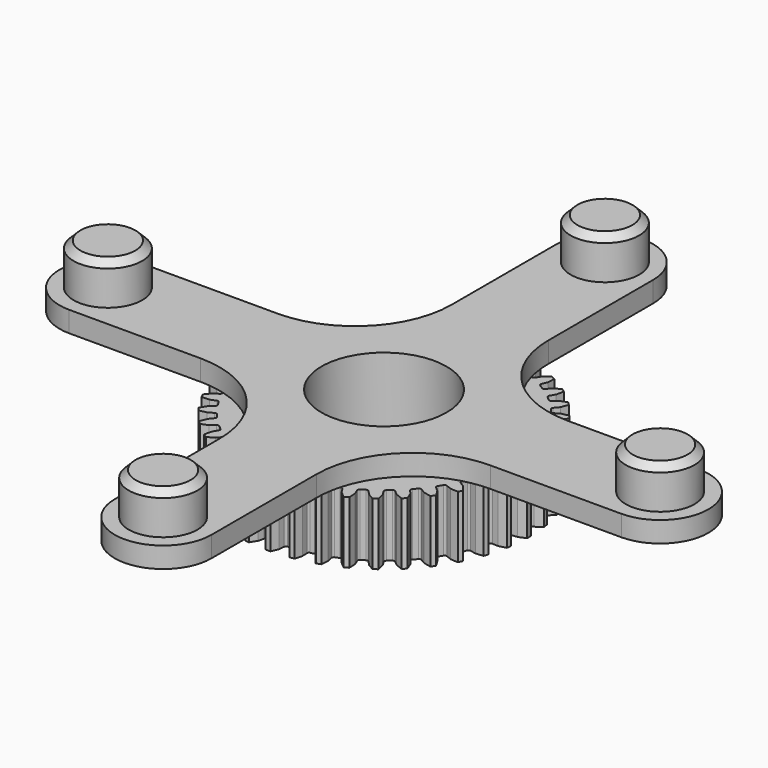
from build123d import *
from build123d import SkipClean  # not in build123d's __all__

# Parameters (mm, degrees)
F0_R     = 4.975
F0_R_2   = 14
F0_R_3   = 1
F0_R_4   = 5
F1_DEPTH = 3
F2_DEPTH = 9
F3_SIZE  = 1
F5_DEPTH = 9
F6_R     = 9.05
F6_R_2   = 5
F7_DEPTH = 18.001


# Not quite as in the source:
# - ends of sketch curves that miss each other by under 0.0002 mm in the source are joined


with BuildPart() as f1:
    # F0 (on Top) → F1 (new body)
    with BuildSketch(Plane.XY):
        with BuildLine():
            ThreePointArc((7, 40.000000175), (-1.75e-07, 47), (-7, 39.999999825))
            Line((-7, 39.999999825), (-6.999999525, 20.9999983))
            ThreePointArc((-6.999999525, 20.9999983), (-11.1005042172, 11.1005033846), (-20.999998825, 6.99999795))
            Line((-20.999998825, 6.99999795), (-40.00000035, 6.999997))
            ThreePointArc((-40.00000035, 6.999997), (-47, -3.35e-06), (-39.99999965, -7.000003))
            Line((-39.99999965, -7.000003), (-20.999999175, -7.00000205))
            ThreePointArc((-20.999999175, -7.00000205), (-11.1005039096, -11.1005067422), (-6.999998475, -21.0000017))
            Line((-6.999998475, -21.0000017), (-6.999998, -40.000000175))
            ThreePointArc((-6.999998, -40.000000175), (2.175e-06, -47), (7.000002, -39.999999825))
            Line((7.000002, -39.999999825), (7.000001525, -21.0000003))
            ThreePointArc((7.000001525, -21.0000003), (11.1005062172, -11.1005053846), (21.000000825, -6.99999995))
            Line((21.000000825, -6.99999995), (40.00000035, -6.999999))
            ThreePointArc((40.00000035, -6.999999), (47, 1.35e-06), (39.99999965, 7.000001))
            Line((39.99999965, 7.000001), (21.000001175, 7.00000005))
            ThreePointArc((21.000001175, 7.00000005), (11.1005059096, 11.1005047422), (7.000000475, 20.9999997))
            Line((7.000000475, 20.9999997), (7, 40.000000175))
        make_face()
        with Locations((-40, -3e-06)):
            Circle(F0_R, mode=Mode.SUBTRACT)
        with Locations((2e-06, -40)):
            Circle(F0_R, mode=Mode.SUBTRACT)
        Circle(F0_R_2, mode=Mode.SUBTRACT)
        with Locations((40, 1e-06)):
            Circle(F0_R, mode=Mode.SUBTRACT)
        with Locations((0, 40)):
            Circle(F0_R, mode=Mode.SUBTRACT)
        with Locations((-40, -3e-06)):
            Circle(F0_R)
        with Locations((-40, -3e-06)):
            Circle(F0_R_3, mode=Mode.SUBTRACT)
        Circle(F0_R_2)
        Circle(F0_R_4, mode=Mode.SUBTRACT)
        with Locations((40, 1e-06)):
            Circle(F0_R)
        with Locations((40, 1e-06)):
            Circle(F0_R_3, mode=Mode.SUBTRACT)
        with Locations((0, 40)):
            Circle(F0_R)
        with Locations((0, 40)):
            Circle(F0_R_3, mode=Mode.SUBTRACT)
        with Locations((2e-06, -40)):
            Circle(F0_R)
        with Locations((2e-06, -40)):
            Circle(F0_R_3, mode=Mode.SUBTRACT)
        with Locations((-40, -3e-06)):
            Circle(F0_R_3)
        with Locations((2e-06, -40)):
            Circle(F0_R_3)
        with Locations((40, 1e-06)):
            Circle(F0_R_3)
        with Locations((0, 40)):
            Circle(F0_R_3)
    extrude(amount=F1_DEPTH)

    # F0 (on Top) → F2 (join)
    with BuildSketch(Plane.XY):
        with Locations((-40, -3e-06)):
            Circle(F0_R)
        with Locations((-40, -3e-06)):
            Circle(F0_R_3, mode=Mode.SUBTRACT)
        with Locations((2e-06, -40)):
            Circle(F0_R)
        with Locations((2e-06, -40)):
            Circle(F0_R_3, mode=Mode.SUBTRACT)
        with Locations((40, 1e-06)):
            Circle(F0_R)
        with Locations((40, 1e-06)):
            Circle(F0_R_3, mode=Mode.SUBTRACT)
        with Locations((0, 40)):
            Circle(F0_R)
        with Locations((0, 40)):
            Circle(F0_R_3, mode=Mode.SUBTRACT)
        with Locations((-40, -3e-06)):
            Circle(F0_R_3)
        with Locations((2e-06, -40)):
            Circle(F0_R_3)
        with Locations((40, 1e-06)):
            Circle(F0_R_3)
        with Locations((0, 40)):
            Circle(F0_R_3)
    extrude(amount=F2_DEPTH)

    # F3
    f3_edges = [f1.edges().sort_by_distance(p)[0] for p in [
        (-44.975, -3e-06, 9),
        (-4.975, 40, 9),
        (35.025, 1e-06, 9),
        (-4.974998, -40, 9),
    ]]
    chamfer(f3_edges, length=F3_SIZE)

    # F4 (on face) → F5 (join)
    with BuildSketch(Plane(origin=(0, 0, 0), x_dir=(1, 0, 0), z_dir=(0, 0, -1))):
        with BuildLine():
            ThreePointArc((7.482641328, 17.3556929783), (11.1005062172, 11.1005053846), (17.3556935395, 7.4826400263))
            ThreePointArc((17.3556935395, 7.4826400263), (17.3405703168, 7.5176207065), (17.3253765901, 7.5525708213))
            ThreePointArc((17.3253765901, 7.5525708213), (17.313509364, 7.760210144), (17.4395229912, 7.9256730139))
            Line((17.4395229912, 7.9256730139), (18.158589, 8.38246))
            Line((18.158589, 8.38246), (18.860183, 9.235448))
            ThreePointArc((18.860183, 9.235448), (18.7111361006, 9.5338022753), (18.557366741, 9.8297578628))
            Line((18.557366741, 9.8297578628), (17.454904, 9.763521))
            Line((17.454904, 9.763521), (16.662699, 9.450277))
            ThreePointArc((16.662699, 9.450277), (16.4547675314, 9.4455858794), (16.2937556703, 9.5772398062))
            ThreePointArc((16.2937556703, 9.5772398062), (16.1149012303, 9.8752194071), (15.9305966906, 10.1698618025))
            ThreePointArc((15.9305966906, 10.1698618025), (15.8863870736, 10.3730992199), (15.9849650752, 10.5562379148))
            Line((15.9849650752, 10.5562379148), (16.623721, 11.119888))
            Line((16.623721, 11.119888), (17.183241, 12.072126))
            ThreePointArc((17.183241, 12.072126), (16.9893574176, 12.3434895607), (16.7911900572, 12.6117380429))
            Line((16.7911900572, 12.6117380429), (15.712654, 12.373864))
            Line((15.712654, 12.373864), (14.979205, 11.940548))
            ThreePointArc((14.979205, 11.940548), (14.7745668627, 11.903388278), (14.5949422111, 12.0082331737))
            ThreePointArc((14.5949422111, 12.0082331737), (14.3716706288, 12.2745705968), (14.1435428129, 12.5367538342))
            ThreePointArc((14.1435428129, 12.5367538342), (14.0680887526, 12.7305673443), (14.1368039213, 12.9268720651))
            Line((14.1368039213, 12.9268720651), (14.679522, 13.583506))
            Line((14.679522, 13.583506), (15.08319, 14.61155))
            ThreePointArc((15.08319, 14.61155), (14.8492371516, 14.8492476582), (14.6115462057, 15.0831932123))
            Line((14.6115462057, 15.0831932123), (13.583506, 14.679522))
            Line((13.583506, 14.679522), (12.926872, 14.136804))
            ThreePointArc((12.926872, 14.136804), (12.7305673443, 14.0680887526), (12.5367531183, 14.1435431335))
            ThreePointArc((12.5367531183, 14.1435431335), (12.2745678752, 14.3716729533), (12.0082271073, 14.5949471304))
            ThreePointArc((12.0082271073, 14.5949471304), (11.9033883527, 14.7745664387), (11.9405484254, 14.9792037487))
            Line((11.9405484254, 14.9792037487), (12.373864, 15.712654))
            Line((12.373864, 15.712654), (12.611741, 16.791188))
            ThreePointArc((12.611741, 16.791188), (12.3434953892, 16.989353183), (12.0721337434, 17.1832356348))
            Line((12.0721337434, 17.1832356348), (11.119888, 16.623721))
            Line((11.119888, 16.623721), (10.556238, 15.984965))
            ThreePointArc((10.556238, 15.984965), (10.3730992199, 15.8863870736), (10.1698673552, 15.9305935563))
            ThreePointArc((10.1698673552, 15.9305935563), (9.8752246071, 16.1148980437), (9.5772429612, 16.293753934))
            ThreePointArc((9.5772429612, 16.293753934), (9.4455858794, 16.4547675314), (9.4502765252, 16.6626991877))
            Line((9.4502765252, 16.6626991877), (9.763521, 17.454904))
            Line((9.763521, 17.454904), (9.829749, 18.557372))
            ThreePointArc((9.829749, 18.557372), (9.5337988946, 18.7111378232), (9.2354479733, 18.8601829454))
            Line((9.2354479733, 18.8601829454), (8.38246, 18.158589))
            Line((8.38246, 18.158589), (7.925673, 17.439523))
            ThreePointArc((7.925673, 17.439523), (7.760210144, 17.313509364), (7.552564996, 17.3253789908))
            ThreePointArc((7.552564996, 17.3253789908), (7.5176153939, 17.34057262), (7.482641328, 17.3556929783))
        make_face()
        with BuildLine():
            ThreePointArc((17.3253765901, -7.5525708213), (17.3405703617, -7.5176206031), (17.3556936288, -7.4826398191))
            ThreePointArc((17.3556936288, -7.4826398191), (11.1005054382, -11.1005052136), (7.4826401704, -17.3556934774))
            ThreePointArc((7.4826401704, -17.3556934774), (7.5176148156, -17.3405728707), (7.552558906, -17.3253817843))
            ThreePointArc((7.552558906, -17.3253817843), (7.7602105823, -17.3135094981), (7.9256730139, -17.4395229912))
            Line((7.9256730139, -17.4395229912), (8.38246, -18.158589))
            Line((8.38246, -18.158589), (9.235448, -18.860183))
            ThreePointArc((9.235448, -18.860183), (9.5337988946, -18.7111378232), (9.8297452293, -18.5573734329))
            Line((9.8297452293, -18.5573734329), (9.763521, -17.454904))
            Line((9.763521, -17.454904), (9.450277, -16.662699))
            ThreePointArc((9.450277, -16.662699), (9.4455858794, -16.4547675314), (9.5772398062, -16.2937556703))
            ThreePointArc((9.5772398062, -16.2937556703), (9.8752246071, -16.1148980437), (10.169867169, -15.9305932647))
            ThreePointArc((10.169867169, -15.9305932647), (10.3730992199, -15.8863870736), (10.5562379148, -15.9849650752))
            Line((10.5562379148, -15.9849650752), (11.119888, -16.623721))
            Line((11.119888, -16.623721), (12.072126, -17.183241))
            ThreePointArc((12.072126, -17.183241), (12.3434953892, -16.989353183), (12.6117437997, -16.7911857333))
            Line((12.6117437997, -16.7911857333), (12.373864, -15.712654))
            Line((12.373864, -15.712654), (11.940548, -14.979205))
            ThreePointArc((11.940548, -14.979205), (11.9033883527, -14.7745664387), (12.0082331737, -14.5949422111))
            ThreePointArc((12.0082331737, -14.5949422111), (12.2745678752, -14.3716729533), (12.5367580597, -14.1435390674))
            ThreePointArc((12.5367580597, -14.1435390674), (12.7305673443, -14.0680887526), (12.9268720651, -14.1368039213))
            Line((12.9268720651, -14.1368039213), (13.583506, -14.679522))
            Line((13.583506, -14.679522), (14.61155, -15.08319))
            ThreePointArc((14.61155, -15.08319), (14.8492371516, -14.8492476582), (15.0831828739, -14.6115568778))
            Line((15.0831828739, -14.6115568778), (14.679522, -13.583506))
            Line((14.679522, -13.583506), (14.136804, -12.926872))
            ThreePointArc((14.136804, -12.926872), (14.0680887526, -12.7305673443), (14.1435431335, -12.5367531183))
            ThreePointArc((14.1435431335, -12.5367531183), (14.3716706288, -12.2745705968), (14.5949389946, -12.0082369956))
            ThreePointArc((14.5949389946, -12.0082369956), (14.7745668627, -11.903388278), (14.9792044899, -11.9405488634))
            Line((14.9792044899, -11.9405488634), (15.712654, -12.373864))
            Line((15.712654, -12.373864), (16.791188, -12.611741))
            ThreePointArc((16.791188, -12.611741), (16.9893574176, -12.3434895607), (17.183239779, -12.0721278447))
            Line((17.183239779, -12.0721278447), (16.623721, -11.119888))
            Line((16.623721, -11.119888), (15.984965, -10.556238))
            ThreePointArc((15.984965, -10.556238), (15.8863870736, -10.3730992199), (15.9305935563, -10.1698673552))
            ThreePointArc((15.9305935563, -10.1698673552), (16.1149012303, -9.8752194071), (16.2937568886, -9.5772379345))
            ThreePointArc((16.2937568886, -9.5772379345), (16.4547675314, -9.4455858794), (16.6626991877, -9.4502765252))
            Line((16.6626991877, -9.4502765252), (17.454904, -9.763521))
            Line((17.454904, -9.763521), (18.557372, -9.829749))
            ThreePointArc((18.557372, -9.829749), (18.7111361006, -9.5338022753), (18.8601858954, -9.2354419488))
            Line((18.8601858954, -9.2354419488), (18.158589, -8.38246))
            Line((18.158589, -8.38246), (17.439523, -7.925673))
            ThreePointArc((17.439523, -7.925673), (17.313509364, -7.760210144), (17.3253765901, -7.5525708213))
        make_face()
        with BuildLine():
            ThreePointArc((-7.5525650468, -17.3253791074), (-7.5176170317, -17.34057191), (-7.4826384548, -17.355694217))
            ThreePointArc((-7.4826384548, -17.355694217), (-11.1005042172, -11.1005033846), (-17.3556947782, -7.4826371531))
            ThreePointArc((-17.3556947782, -7.4826371531), (-17.3405721919, -7.5176163814), (-17.3253791074, -7.5525650468))
            ThreePointArc((-17.3253791074, -7.5525650468), (-17.3135094981, -7.7602105823), (-17.4395229912, -7.9256730139))
            Line((-17.4395229912, -7.9256730139), (-18.158589, -8.38246))
            Line((-18.158589, -8.38246), (-18.860183, -9.235448))
            ThreePointArc((-18.860183, -9.235448), (-18.7111345743, -9.5338052708), (-18.5573702937, -9.8297511556))
            Line((-18.5573702937, -9.8297511556), (-17.454904, -9.763521))
            Line((-17.454904, -9.763521), (-16.662699, -9.450277))
            ThreePointArc((-16.662699, -9.450277), (-16.454767939, -9.4455857391), (-16.2937561071, -9.577239063))
            ThreePointArc((-16.2937561071, -9.577239063), (-16.1148997927, -9.875221753), (-15.9305901283, -10.1698720819))
            ThreePointArc((-15.9305901283, -10.1698720819), (-15.8863870736, -10.3730992199), (-15.9849650752, -10.5562379148))
            Line((-15.9849650752, -10.5562379148), (-16.623721, -11.119888))
            Line((-16.623721, -11.119888), (-17.183241, -12.072126))
            ThreePointArc((-17.183241, -12.072126), (-16.9893616522, -12.3434837323), (-16.791194381, -12.6117322862))
            Line((-16.791194381, -12.6117322862), (-15.712654, -12.373864))
            Line((-15.712654, -12.373864), (-14.979205, -11.940548))
            ThreePointArc((-14.979205, -11.940548), (-14.7745667516, -11.9033882976), (-14.5949426148, -12.008232683))
            ThreePointArc((-14.5949426148, -12.008232683), (-14.3716752415, -12.274565196), (-14.1435470548, -12.5367490486))
            ThreePointArc((-14.1435470548, -12.5367490486), (-14.0680887526, -12.7305673443), (-14.1368039213, -12.9268720651))
            Line((-14.1368039213, -12.9268720651), (-14.679522, -13.583506))
            Line((-14.679522, -13.583506), (-15.08319, -14.61155))
            ThreePointArc((-15.08319, -14.61155), (-14.8492426589, -14.849242151), (-14.6115517997, -15.0831877932))
            Line((-14.6115517997, -15.0831877932), (-13.583506, -14.679522))
            Line((-13.583506, -14.679522), (-12.926872, -14.136804))
            ThreePointArc((-12.926872, -14.136804), (-12.7305670127, -14.0680887583), (-12.5367526219, -14.1435435735))
            ThreePointArc((-12.5367526219, -14.1435435735), (-12.2745657312, -14.3716747845), (-12.0082320514, -14.5949430625))
            ThreePointArc((-12.0082320514, -14.5949430625), (-11.903388278, -14.7745668627), (-11.9405488634, -14.9792044899))
            Line((-11.9405488634, -14.9792044899), (-12.373864, -15.712654))
            Line((-12.373864, -15.712654), (-12.611741, -16.791188))
            ThreePointArc((-12.611741, -16.791188), (-12.3434840557, -16.9893614172), (-12.072121946, -17.1832439231))
            Line((-12.072121946, -17.1832439231), (-11.119888, -16.623721))
            Line((-11.119888, -16.623721), (-10.556238, -15.984965))
            ThreePointArc((-10.556238, -15.984965), (-10.3730992199, -15.8863870736), (-10.1698673552, -15.9305935563))
            ThreePointArc((-10.1698673552, -15.9305935563), (-9.8752221123, -16.1148995725), (-9.5772321646, -16.2937602801))
            ThreePointArc((-9.5772321646, -16.2937602801), (-9.4455857391, -16.454767939), (-9.4502765252, -16.6626991877))
            Line((-9.4502765252, -16.6626991877), (-9.763521, -17.454904))
            Line((-9.763521, -17.454904), (-9.829749, -18.557372))
            ThreePointArc((-9.829749, -18.557372), (-9.5338056645, -18.7111343737), (-9.2354548043, -18.8601796004))
            Line((-9.2354548043, -18.8601796004), (-8.38246, -18.158589))
            Line((-8.38246, -18.158589), (-7.925673, -17.439523))
            ThreePointArc((-7.925673, -17.439523), (-7.760210144, -17.313509364), (-7.5525650468, -17.3253791074))
        make_face()
        with BuildLine():
            ThreePointArc((-17.3556929162, 7.4826414721), (-11.100504381, 11.1005062708), (-7.4826385175, 17.35569419))
            ThreePointArc((-7.4826385175, 17.35569419), (-7.517617063, 17.3405718964), (-7.5525650468, 17.3253791074))
            ThreePointArc((-7.5525650468, 17.3253791074), (-7.7602105823, 17.3135094981), (-7.9256730139, 17.4395229912))
            Line((-7.9256730139, 17.4395229912), (-8.38246, 18.158589))
            Line((-8.38246, 18.158589), (-9.235448, 18.860183))
            ThreePointArc((-9.235448, 18.860183), (-9.5338056645, 18.7111343737), (-9.8297519365, 18.5573698801))
            Line((-9.8297519365, 18.5573698801), (-9.763521, 17.454904))
            Line((-9.763521, 17.454904), (-9.450277, 16.662699))
            ThreePointArc((-9.450277, 16.662699), (-9.4455857391, 16.454767939), (-9.577239063, 16.2937561071))
            ThreePointArc((-9.577239063, 16.2937561071), (-9.8752221123, 16.1148995725), (-10.1698727924, 15.9305896748))
            ThreePointArc((-10.1698727924, 15.9305896748), (-10.3730992199, 15.8863870736), (-10.5562379148, 15.9849650752))
            Line((-10.5562379148, 15.9849650752), (-11.119888, 16.623721))
            Line((-11.119888, 16.623721), (-12.072126, 17.183241))
            ThreePointArc((-12.072126, 17.183241), (-12.3434840557, 16.9893614172), (-12.6117329255, 16.7911939008))
            Line((-12.6117329255, 16.7911939008), (-12.373864, 15.712654))
            Line((-12.373864, 15.712654), (-11.940548, 14.979205))
            ThreePointArc((-11.940548, 14.979205), (-11.903388278, 14.7745668627), (-12.0082331737, 14.5949422111))
            ThreePointArc((-12.0082331737, 14.5949422111), (-12.2745657312, 14.3716747845), (-12.5367490486, 14.1435470548))
            ThreePointArc((-12.5367490486, 14.1435470548), (-12.7305670127, 14.0680887583), (-12.9268720651, 14.1368039213))
            Line((-12.9268720651, 14.1368039213), (-13.583506, 14.679522))
            Line((-13.583506, 14.679522), (-14.61155, 15.08319))
            ThreePointArc((-14.61155, 15.08319), (-14.8492426589, 14.849242151), (-15.083188293, 14.6115512838))
            Line((-15.083188293, 14.6115512838), (-14.679522, 13.583506))
            Line((-14.679522, 13.583506), (-14.136804, 12.926872))
            ThreePointArc((-14.136804, 12.926872), (-14.0680887583, 12.7305670127), (-14.1435435735, 12.5367526219))
            ThreePointArc((-14.1435435735, 12.5367526219), (-14.3716752415, 12.274565196), (-14.5949439568, 12.0082309645))
            ThreePointArc((-14.5949439568, 12.0082309645), (-14.7745667516, 11.9033882976), (-14.9792037487, 11.9405484254))
            Line((-14.9792037487, 11.9405484254), (-15.712654, 12.373864))
            Line((-15.712654, 12.373864), (-16.791188, 12.611741))
            ThreePointArc((-16.791188, 12.611741), (-16.9893616522, 12.3434837323), (-17.1832439231, 12.072121946))
            Line((-17.1832439231, 12.072121946), (-16.623721, 11.119888))
            Line((-16.623721, 11.119888), (-15.984965, 10.556238))
            ThreePointArc((-15.984965, 10.556238), (-15.8863870736, 10.3730992199), (-15.9305935563, 10.1698673552))
            ThreePointArc((-15.9305935563, 10.1698673552), (-16.1148997927, 9.875221753), (-16.2937602801, 9.5772321646))
            ThreePointArc((-16.2937602801, 9.5772321646), (-16.454767939, 9.4455857391), (-16.6626991877, 9.4502765252))
            Line((-16.6626991877, 9.4502765252), (-17.454904, 9.763521))
            Line((-17.454904, 9.763521), (-18.557372, 9.829749))
            ThreePointArc((-18.557372, 9.829749), (-18.7111345743, 9.5338052708), (-18.8601796004, 9.2354548043))
            Line((-18.8601796004, 9.2354548043), (-18.158589, 8.38246))
            Line((-18.158589, 8.38246), (-17.439523, 7.925673))
            ThreePointArc((-17.439523, 7.925673), (-17.313509364, 7.760210144), (-17.3253789908, 7.552564996))
            ThreePointArc((-17.3253789908, 7.552564996), (-17.3405712565, 7.517618539), (-17.3556929162, 7.4826414721))
        make_face()
        with BuildLine():
            Line((19.984979, -0.775), (20.997352, -0.3335))
            ThreePointArc((20.997352, -0.3335), (20.9993378789, -0.1667592543), (21, 0))
            ThreePointArc((21, 0), (20.9993378789, 0.1667592543), (20.9973515572, 0.333507993))
            Line((20.9973515572, 0.333507993), (19.984979, 0.775))
            Line((19.984979, 0.775), (19.136909, 0.855551))
            ThreePointArc((19.136909, 0.855551), (18.9495117324, 0.9457704849), (18.8658185942, 1.1361719756))
            ThreePointArc((18.8658185942, 1.1361719756), (18.841738095, 1.4828707153), (18.8112863856, 1.8290720375))
            ThreePointArc((18.8112863856, 1.8290720375), (18.864162521, 2.0302303867), (19.0351398721, 2.1486544974))
            Line((19.0351398721, 2.1486544974), (19.860167, 2.360881))
            Line((19.860167, 2.360881), (20.79101, 2.955315))
            ThreePointArc((20.79101, 2.955315), (20.741455614, 3.2851208523), (20.6866695003, 3.6140980874))
            Line((20.6866695003, 3.6140980874), (19.617694, 3.891798))
            Line((19.617694, 3.891798), (18.767464, 3.83869))
            ThreePointArc((18.767464, 3.83869), (18.5682605457, 3.8984829106), (18.455812421, 4.0734488722))
            ThreePointArc((18.455812421, 4.0734488722), (18.3777913721, 4.4121178911), (18.2935567001, 4.7492929221))
            ThreePointArc((18.2935567001, 4.7492929221), (18.3143156741, 4.9562403103), (18.4646620532, 5.0999528771))
            Line((18.4646620532, 5.0999528771), (19.246332, 5.438629))
            Line((19.246332, 5.438629), (20.072725, 6.171361))
            ThreePointArc((20.072725, 6.171361), (19.9721853646, 6.4893614296), (19.8666102165, 6.8057180742))
            Line((19.8666102165, 6.8057180742), (18.767356, 6.912767))
            Line((18.767356, 6.912767), (17.935902, 6.727308))
            ThreePointArc((17.935902, 6.727308), (17.7297970592, 6.7552024565), (17.5913629266, 6.9104229712))
            ThreePointArc((17.5913629266, 6.9104229712), (17.4758722837, 7.1974917799), (17.3556935395, 7.4826400263))
            ThreePointArc((17.3556935395, 7.4826400263), (11.1005062172, 11.1005053846), (7.482641328, 17.3556929783))
            ThreePointArc((7.482641328, 17.3556929783), (7.1974953552, 17.4758708112), (6.9104200778, 17.591364198))
            ThreePointArc((6.9104200778, 17.591364198), (6.7552024565, 17.7297970592), (6.7273075269, 17.9359021055))
            Line((6.7273075269, 17.9359021055), (6.912767, 18.767356))
            Line((6.912767, 18.767356), (6.805716, 19.866611))
            ThreePointArc((6.805716, 19.866611), (6.489358419, 19.9721863428), (6.1713550577, 20.0727271877))
            Line((6.1713550577, 20.0727271877), (5.438629, 19.246332))
            Line((5.438629, 19.246332), (5.099953, 18.464662))
            ThreePointArc((5.099953, 18.464662), (4.9562398754, 18.3143154618), (4.7492940456, 18.2935561756))
            ThreePointArc((4.7492940456, 18.2935561756), (4.4121239122, 18.3777899265), (4.0734569339, 18.4558107004))
            ThreePointArc((4.0734569339, 18.4558107004), (3.8984832108, 18.5682601471), (3.8386895107, 18.7674640306))
            Line((3.8386895107, 18.7674640306), (3.891798, 19.617694))
            Line((3.891798, 19.617694), (3.614104, 20.686669))
            ThreePointArc((3.614104, 20.686669), (3.2851278346, 20.7414545081), (2.9553220557, 20.7910093922))
            Line((2.9553220557, 20.7910093922), (2.360881, 19.860167))
            Line((2.360881, 19.860167), (2.148654, 19.03514))
            ThreePointArc((2.148654, 19.03514), (2.0302303867, 18.864162521), (1.8290799194, 18.8112851712))
            ThreePointArc((1.8290799194, 18.8112851712), (1.4828772049, 18.8417375843), (1.1361750279, 18.8658184637))
            ThreePointArc((1.1361750279, 18.8658184637), (0.9457704849, 18.9495117324), (0.8555511543, 19.1369090147))
            Line((0.8555511543, 19.1369090147), (0.775, 19.984979))
            Line((0.775, 19.984979), (0.3335, 20.997352))
            ThreePointArc((0.3335, 20.997352), (-3.4996e-06, 21), (-0.3335009947, 20.9973516684))
            Line((-0.3335009947, 20.9973516684), (-0.775, 19.984979))
            Line((-0.775, 19.984979), (-0.855551, 19.136909))
            ThreePointArc((-0.855551, 19.136909), (-0.9457704849, 18.9495117324), (-1.1361719756, 18.8658185942))
            ThreePointArc((-1.1361719756, 18.8658185942), (-1.4828837113, 18.8417370722), (-1.8290850121, 18.8112851241))
            ThreePointArc((-1.8290850121, 18.8112851241), (-2.0302303867, 18.864162521), (-2.1486544974, 19.0351398721))
            Line((-2.1486544974, 19.0351398721), (-2.360881, 19.860167))
            Line((-2.360881, 19.860167), (-2.955315, 20.79101))
            ThreePointArc((-2.955315, 20.79101), (-3.2851243409, 20.7414550614), (-3.6141120118, 20.6866670676))
            Line((-3.6141120118, 20.6866670676), (-3.891798, 19.617694))
            Line((-3.891798, 19.617694), (-3.83869, 18.767464))
            ThreePointArc((-3.83869, 18.767464), (-3.8984829171, 18.5682605371), (-4.0734479187, 18.4558126315))
            ThreePointArc((-4.0734479187, 18.4558126315), (-4.412111992, 18.3777927883), (-4.7492870578, 18.2935582226))
            ThreePointArc((-4.7492870578, 18.2935582226), (-4.9562403103, 18.3143156741), (-5.0999528771, 18.4646620532))
            Line((-5.0999528771, 18.4646620532), (-5.438629, 19.246332))
            Line((-5.438629, 19.246332), (-6.171361, 20.072725))
            ThreePointArc((-6.171361, 20.072725), (-6.4893554155, 19.9721873186), (-6.8057120912, 19.8666122661))
            Line((-6.8057120912, 19.8666122661), (-6.912767, 18.767356))
            Line((-6.912767, 18.767356), (-6.727308, 17.935902))
            ThreePointArc((-6.727308, 17.935902), (-6.7552022275, 17.7297974901), (-6.9104229712, 17.5913629266))
            ThreePointArc((-6.9104229712, 17.5913629266), (-7.1974968602, 17.4758701914), (-7.4826385175, 17.35569419))
            ThreePointArc((-7.4826385175, 17.35569419), (-11.100504381, 11.1005062708), (-17.3556929162, 7.4826414721))
            ThreePointArc((-17.3556929162, 7.4826414721), (-17.4758695788, 7.1974983477), (-17.5913618888, 6.9104259563))
            ThreePointArc((-17.5913618888, 6.9104259563), (-17.7297970592, 6.7552024565), (-17.9359021055, 6.7273075269))
            Line((-17.9359021055, 6.7273075269), (-18.767356, 6.912767))
            Line((-18.767356, 6.912767), (-19.866611, 6.805716))
            ThreePointArc((-19.866611, 6.805716), (-19.9721876626, 6.489354357), (-20.0727253296, 6.1713611013))
            Line((-20.0727253296, 6.1713611013), (-19.246332, 5.438629))
            Line((-19.246332, 5.438629), (-18.464662, 5.099953))
            ThreePointArc((-18.464662, 5.099953), (-18.3143154618, 4.9562398754), (-18.2935561756, 4.7492940456))
            ThreePointArc((-18.2935561756, 4.7492940456), (-18.3777927883, 4.412111992), (-18.4558133188, 4.0734450704))
            ThreePointArc((-18.4558133188, 4.0734450704), (-18.5682605371, 3.8984829171), (-18.7674640306, 3.8386895107))
            Line((-18.7674640306, 3.8386895107), (-19.617694, 3.891798))
            Line((-19.617694, 3.891798), (-20.686669, 3.614104))
            ThreePointArc((-20.686669, 3.614104), (-20.7414550614, 3.2851243409), (-20.7910113824, 2.9553080544))
            Line((-20.7910113824, 2.9553080544), (-19.860167, 2.360881))
            Line((-19.860167, 2.360881), (-19.03514, 2.148654))
            ThreePointArc((-19.03514, 2.148654), (-18.864162521, 2.0302303867), (-18.8112851712, 1.8290799194))
            ThreePointArc((-18.8112851712, 1.8290799194), (-18.8417371113, 1.4828832152), (-18.8658181037, 1.1361810062))
            ThreePointArc((-18.8658181037, 1.1361810062), (-18.9495117324, 0.9457704849), (-19.1369090147, 0.8555511543))
            Line((-19.1369090147, 0.8555511543), (-19.984979, 0.775))
            Line((-19.984979, 0.775), (-20.997352, 0.3335))
            ThreePointArc((-20.997352, 0.3335), (-20.9993379345, 0.166752255), (-21, -7e-06))
            ThreePointArc((-21, -7e-06), (-20.9993378789, -0.1667592548), (-20.9973516684, -0.3335009947))
            Line((-20.9973516684, -0.3335009947), (-19.984979, -0.775))
            Line((-19.984979, -0.775), (-19.136909, -0.855551))
            ThreePointArc((-19.136909, -0.855551), (-18.9495117324, -0.9457704849), (-18.8658185942, -1.1361719756))
            ThreePointArc((-18.8658185942, -1.1361719756), (-18.8417371113, -1.4828832152), (-18.8112852204, -1.8290840214))
            ThreePointArc((-18.8112852204, -1.8290840214), (-18.864162521, -2.0302303867), (-19.0351398721, -2.1486544974))
            Line((-19.0351398721, -2.1486544974), (-19.860167, -2.360881))
            Line((-19.860167, -2.360881), (-20.79101, -2.955315))
            ThreePointArc((-20.79101, -2.955315), (-20.7414550614, -3.2851243409), (-20.6866670676, -3.6141120118))
            Line((-20.6866670676, -3.6141120118), (-19.617694, -3.891798))
            Line((-19.617694, -3.891798), (-18.767464, -3.83869))
            ThreePointArc((-18.767464, -3.83869), (-18.5682605371, -3.8984829171), (-18.4558126315, -4.0734479187))
            ThreePointArc((-18.4558126315, -4.0734479187), (-18.3777927883, -4.412111992), (-18.2935582226, -4.7492870578))
            ThreePointArc((-18.2935582226, -4.7492870578), (-18.3143154618, -4.9562398754), (-18.4646620532, -5.0999528771))
            Line((-18.4646620532, -5.0999528771), (-19.246332, -5.438629))
            Line((-19.246332, -5.438629), (-20.072725, -6.171361))
            ThreePointArc((-20.072725, -6.171361), (-19.9721876626, -6.489354357), (-19.8666126777, -6.8057108896))
            Line((-19.8666126777, -6.8057108896), (-18.767356, -6.912767))
            Line((-18.767356, -6.912767), (-17.935902, -6.727308))
            ThreePointArc((-17.935902, -6.727308), (-17.7297970592, -6.7552024565), (-17.5913629266, -6.9104229712))
            ThreePointArc((-17.5913629266, -6.9104229712), (-17.4758704743, -7.1974961733), (-17.3556947782, -7.4826371531))
            ThreePointArc((-17.3556947782, -7.4826371531), (-11.1005042172, -11.1005033846), (-7.4826384548, -17.355694217))
            ThreePointArc((-7.4826384548, -17.355694217), (-7.1974968287, -17.4758702044), (-6.9104259563, -17.5913618888))
            ThreePointArc((-6.9104259563, -17.5913618888), (-6.7552022275, -17.7297974901), (-6.7273077393, -17.9359030581))
            Line((-6.7273077393, -17.9359030581), (-6.912767, -18.767356))
            Line((-6.912767, -18.767356), (-6.805716, -19.866611))
            ThreePointArc((-6.805716, -19.866611), (-6.4893554155, -19.9721873186), (-6.171362015, -20.0727250487))
            Line((-6.171362015, -20.0727250487), (-5.438629, -19.246332))
            Line((-5.438629, -19.246332), (-5.099953, -18.464662))
            ThreePointArc((-5.099953, -18.464662), (-4.9562398754, -18.3143154618), (-4.7492940456, -18.2935561756))
            ThreePointArc((-4.7492940456, -18.2935561756), (-4.412111992, -18.3777927883), (-4.0734450704, -18.4558133188))
            ThreePointArc((-4.0734450704, -18.4558133188), (-3.8984829171, -18.5682605371), (-3.8386895107, -18.7674640306))
            Line((-3.8386895107, -18.7674640306), (-3.891798, -19.617694))
            Line((-3.891798, -19.617694), (-3.614104, -20.686669))
            ThreePointArc((-3.614104, -20.686669), (-3.2851243409, -20.7414550614), (-2.9553080544, -20.7910113824))
            Line((-2.9553080544, -20.7910113824), (-2.360881, -19.860167))
            Line((-2.360881, -19.860167), (-2.148654, -19.03514))
            ThreePointArc((-2.148654, -19.03514), (-2.0302303867, -18.864162521), (-1.8290799194, -18.8112851712))
            ThreePointArc((-1.8290799194, -18.8112851712), (-1.4828837113, -18.8417370722), (-1.1361810062, -18.8658181037))
            ThreePointArc((-1.1361810062, -18.8658181037), (-0.9457704849, -18.9495117324), (-0.8555511543, -19.1369090147))
            Line((-0.8555511543, -19.1369090147), (-0.775, -19.984979))
            Line((-0.775, -19.984979), (-0.3335, -20.997352))
            ThreePointArc((-0.3335, -20.997352), (-3.4996e-06, -21), (0.3334939965, -20.9973517796))
            Line((0.3334939965, -20.9973517796), (0.775, -19.984979))
            Line((0.775, -19.984979), (0.855551, -19.136909))
            ThreePointArc((0.855551, -19.136909), (0.9457704849, -18.9495117324), (1.1361719756, -18.8658185942))
            ThreePointArc((1.1361719756, -18.8658185942), (1.4828772049, -18.8417375843), (1.8290779813, -18.8112858077))
            ThreePointArc((1.8290779813, -18.8112858077), (2.0302303867, -18.864162521), (2.1486544974, -19.0351398721))
            Line((2.1486544974, -19.0351398721), (2.360881, -19.860167))
            Line((2.360881, -19.860167), (2.955315, -20.79101))
            ThreePointArc((2.955315, -20.79101), (3.2851278346, -20.7414545081), (3.6141050496, -20.686668284))
            Line((3.6141050496, -20.686668284), (3.891798, -19.617694))
            Line((3.891798, -19.617694), (3.83869, -18.767464))
            ThreePointArc((3.83869, -18.767464), (3.8984832108, -18.5682601471), (4.0734488722, -18.455812421))
            ThreePointArc((4.0734488722, -18.455812421), (4.4121239122, -18.3777899265), (4.7492990297, -18.2935551145))
            ThreePointArc((4.7492990297, -18.2935551145), (4.9562398754, -18.3143154618), (5.0999528771, -18.4646620532))
            Line((5.0999528771, -18.4646620532), (5.438629, -19.246332))
            Line((5.438629, -19.246332), (6.171361, -20.072725))
            ThreePointArc((6.171361, -20.072725), (6.489358419, -19.9721863428), (6.8057249521, -19.8666078603))
            Line((6.8057249521, -19.8666078603), (6.912767, -18.767356))
            Line((6.912767, -18.767356), (6.727308, -17.935902))
            ThreePointArc((6.727308, -17.935902), (6.7552024565, -17.7297970592), (6.9104229712, -17.5913629266))
            ThreePointArc((6.9104229712, -17.5913629266), (7.1974947724, -17.4758710513), (7.4826401704, -17.3556934774))
            ThreePointArc((7.4826401704, -17.3556934774), (11.1005054382, -11.1005052136), (17.3556936288, -7.4826398191))
            ThreePointArc((17.3556936288, -7.4826398191), (17.4758723267, -7.1974916756), (17.5913665073, -6.9104141993))
            ThreePointArc((17.5913665073, -6.9104141993), (17.7297970592, -6.7552024565), (17.9359021055, -6.7273075269))
            Line((17.9359021055, -6.7273075269), (18.767356, -6.912767))
            Line((18.767356, -6.912767), (19.866611, -6.805716))
            ThreePointArc((19.866611, -6.805716), (19.9721853646, -6.4893614296), (20.0727231906, -6.1713680586))
            Line((20.0727231906, -6.1713680586), (19.246332, -5.438629))
            Line((19.246332, -5.438629), (18.464662, -5.099953))
            ThreePointArc((18.464662, -5.099953), (18.3143154618, -4.9562398754), (18.2935561756, -4.7492940456))
            ThreePointArc((18.2935561756, -4.7492940456), (18.3777913721, -4.4121178911), (18.4558120096, -4.0734510021))
            ThreePointArc((18.4558120096, -4.0734510021), (18.5682609357, -3.8984826168), (18.7674650267, -3.8386895729))
            Line((18.7674650267, -3.8386895729), (19.617694, -3.891798))
            Line((19.617694, -3.891798), (20.686669, -3.614104))
            ThreePointArc((20.686669, -3.614104), (20.741455614, -3.2851208523), (20.7910103873, -2.9553150551))
            Line((20.7910103873, -2.9553150551), (19.860167, -2.360881))
            Line((19.860167, -2.360881), (19.03514, -2.148654))
            ThreePointArc((19.03514, -2.148654), (18.864162521, -2.0302303867), (18.8112851712, -1.8290799194))
            ThreePointArc((18.8112851712, -1.8290799194), (18.841738095, -1.4828707153), (18.8658188874, -1.1361679932))
            ThreePointArc((18.8658188874, -1.1361679932), (18.9495117324, -0.9457704849), (19.1369090147, -0.8555511543))
            Line((19.1369090147, -0.8555511543), (19.984979, -0.775))
        make_face()
        with BuildLine():
            ThreePointArc((12.5, 0), (2e-06, -12.5), (-12.5, -4e-06))
            ThreePointArc((-12.5, -4e-06), (-2e-06, 12.5), (12.5, 0))
        make_face(mode=Mode.SUBTRACT)
        with BuildLine():
            ThreePointArc((12.5, 0), (-2e-06, 12.5), (-12.5, -4e-06))
            ThreePointArc((-12.5, -4e-06), (2e-06, -12.5), (12.5, 0))
        make_face()
        with BuildLine():
            ThreePointArc((5, 0), (3.535534613, -3.5355331988), (2e-06, -5))
            ThreePointArc((2e-06, -5), (-5, 0), (2e-06, 5))
            ThreePointArc((2e-06, 5), (3.535534613, 3.5355331988), (5, 0))
        make_face(mode=Mode.SUBTRACT)
    with SkipClean():  # cleaning this boolean's faces spoils the solid; the shape is the same uncleaned
        extrude(amount=F5_DEPTH)

    # F6 (on face) → F7 (cut, through all)
    with BuildSketch(Plane(origin=(0, 0, -9), x_dir=(1, 0, 0), z_dir=(0, 0, -1))):
        Circle(F6_R)
        Circle(F6_R_2, mode=Mode.SUBTRACT)
    extrude(amount=-F7_DEPTH, mode=Mode.SUBTRACT)


solid = f1.part
